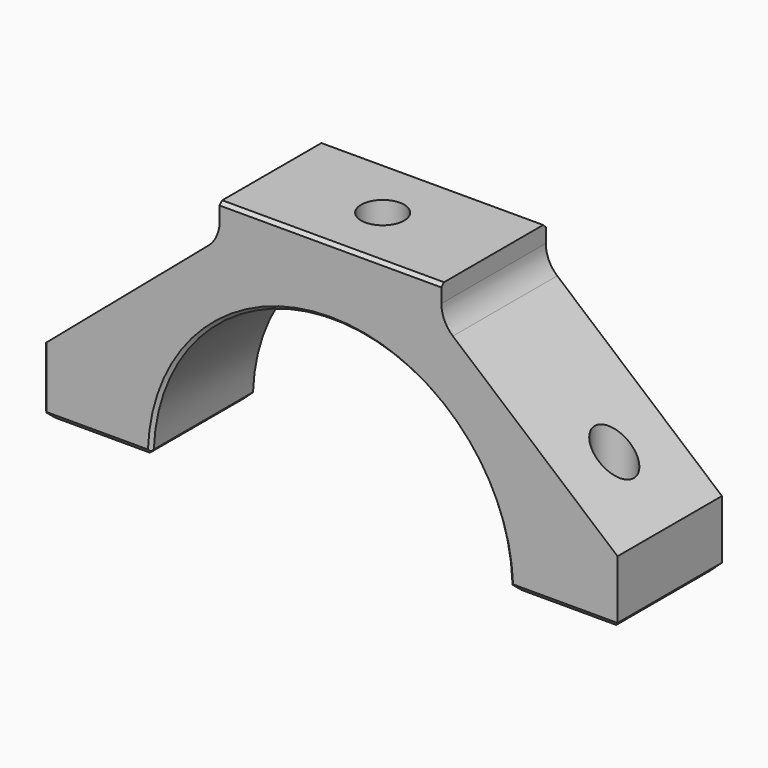
from build123d import *

# Parameters (mm, degrees)
F1_DEPTH    = 20
F3_D        = 6
F4_T1_DEPTH = 21.6433659759
F4_T3_DEPTH = 21.6433659759
F4_T5_DEPTH = 25.0580427678
F4_T7_DEPTH = 25.1433659759
F5_SIZE     = 0.5
F7_D        = 6.6
F9_R        = 5.5
F10_DEPTH   = 3.5
F11_R       = 5


# Not quite as in the source:
# - a fillet or chamfer that OpenCascade refuses, or shapes differently, is made with other operations: its cross-section is extruded or revolved along the edge and cut away or added
# - a feature names something its author has since deleted; it is built from what else it names


with BuildPart() as f1:
    # F0 (on Front) → F1 (new body)
    with BuildSketch(Plane.XZ):
        with BuildLine():
            ThreePointArc((-27.5, 0), (0, 27.5), (27.5, 0))
            Line((27.5, 0), (44, 0))
            Line((44, 0), (44, 10))
            Line((44, 10), (17, 33))
            Line((17, 33), (17, 38))
            Line((17, 38), (-17, 38))
            Line((-17, 38), (-17, 33))
            Line((-17, 33), (-44, 10))
            Line((-44, 10), (-44, 0))
            Line((-44, 0), (-27.5, 0))
        make_face()
    extrude(amount=-F1_DEPTH)

    # F3 (through all)
    with Locations(Plane(origin=(0, 0, 0), x_dir=(1, 0, 0), z_dir=(0, 0, -1))):
        with Locations((-35.5, -10), (35.5, -10)):
            Hole(F3_D / 2)

    # F4: chamfer of 1 on 8 edges, made by hand

    # F4_s2 → F4_t1 (cut)
    with BuildSketch(Plane.YZ.offset(24.928317012)):
        Polygon((19, 0), (20, 1), (20, 0), align=None)
        Polygon((1, 0), (0, 1), (0, 0), align=None)
    extrude(amount=F4_T1_DEPTH, mode=Mode.SUBTRACT)

    # F4_s4 → F4_t3 (cut)
    with BuildSketch(Plane.YZ.offset(-46.571682988)):
        Polygon((19, 0), (20, 1), (20, 0), align=None)
        Polygon((1, 0), (0, 1), (0, 0), align=None)
    extrude(amount=F4_T3_DEPTH, mode=Mode.SUBTRACT)

    # F4_s6 → F4_t5 (cut)
    with BuildSketch(Plane.XZ.offset(-22.5290213839)):
        with BuildLine():
            Line((-27.4830665009, 0.9649122807), (-28.4824507373, 0))
            Line((-28.4824507373, 0), (-27.5, 0))
            ThreePointArc((-27.5, 0), (-27.4955143469, 0.4966797747), (-27.4830665009, 0.9649122807))
        make_face()
        with BuildLine():
            Line((27.4830665009, 0.9649122807), (28.4824507373, 0))
            Line((28.4824507373, 0), (27.5, 0))
            ThreePointArc((27.5, 0), (27.4955143469, 0.4966797747), (27.4830665009, 0.9649122807))
        make_face()
    extrude(amount=F4_T5_DEPTH, mode=Mode.SUBTRACT)

    # F4_s8 → F4_t7 (cut)
    with BuildSketch(Plane.XZ.offset(-22.571682988)):
        Polygon((-43, 0), (-44, 1), (-44, 0), align=None)
        Polygon((43, 0), (44, 1), (44, 0), align=None)
    extrude(amount=F4_T7_DEPTH, mode=Mode.SUBTRACT)

    # F5
    f5_edges = [f1.edges().sort_by_distance(p)[0] for p in [
        (0, 20, 38),
        (0, 0, 38),
        (0, 20, 27.5),
        (-44, 20, 5.5),
        (0, 0, 27.5),
        (-44, 0, 5.5),
    ]]
    chamfer(f5_edges, length=F5_SIZE)

    # F7 (through all)
    with Locations(Plane.XY.offset(38)):
        with Locations((0, 10)):
            Hole(F7_D / 2)

    # F9 (on offset) → F10 (cut, symmetric)
    with BuildSketch(Plane.XY.offset(27.5)):
        with Locations((0, 10)):
            Circle(F9_R)
    extrude(amount=F10_DEPTH, both=True, mode=Mode.SUBTRACT)

    # F11
    f11_edges = [f1.edges().sort_by_distance(p)[0] for p in [
        (-17, 10, 33),
        (17, 10, 33),
    ]]
    fillet(f11_edges, radius=F11_R)


solid = f1.part
